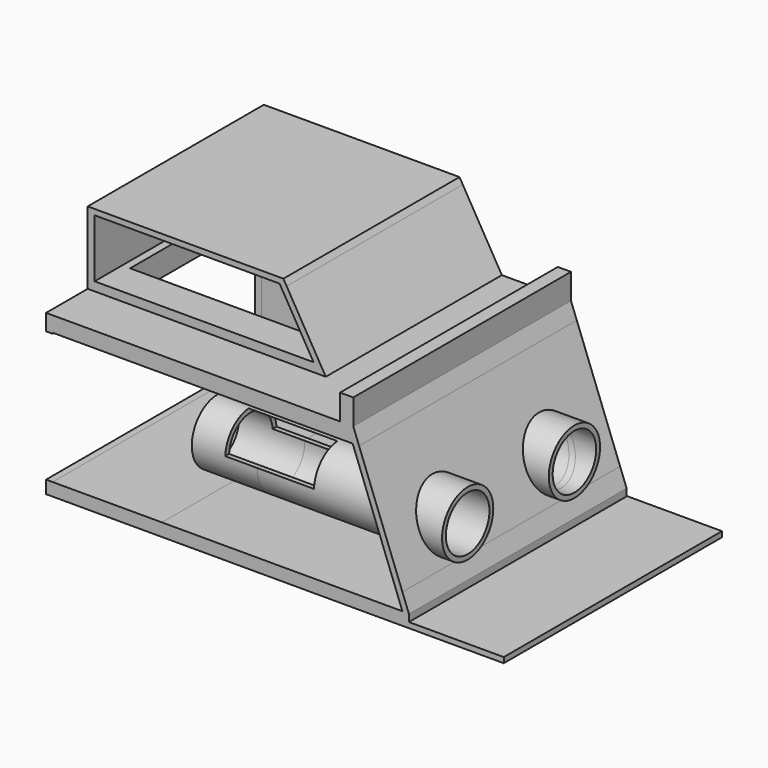
from build123d import *

# Parameters (mm, degrees)
F0_W      = 154.8604735136
F0_H      = 381
F0_W_2    = 202.8337074444
F0_W_3    = 150.305819042
F1_DEPTH  = 215.9
F3_DEPTH  = 365.76
F4_DEPTH  = 474.472
F5_DEPTH  = 384.81
F6_DEPTH  = 463.296
F7_DEPTH  = 453.644
F8_DEPTH  = 401.828
F9_W      = 333.3268084526
F9_H      = 308.1617667079
F10_DEPTH = 101.6
F12_DEPTH = 332.74
F13_DEPTH = 290.83
F14_W     = 640.7658
F14_H     = 381.7952661514
F15_DEPTH = 7.62
F16_W     = 18.4519021228
F16_H     = 174.1818501353
F16_H_2   = 32.6362997293
F17_DEPTH = 35.56
F18_R     = 44.8167953051
F18_R_2   = 38.1
F19_DEPTH = 258.572
F20_DEPTH = 485.14
F21_DEPTH = 258.572
F22_DEPTH = 57.658
F23_DEPTH = 72.898
F24_DEPTH = 250.19
F25_W     = 142.1934430047
F25_H     = 97.1279808664
F26_DEPTH = 68.58
F28_DEPTH = 340.868
F30_W     = 177.6428297162
F30_H     = 182.6925156638
F31_DEPTH = 723.9


# Not quite as in the source:
# - the program builds the solid bodies; features that only make, move or delete a surface that nothing else refers to are left out


with BuildPart() as f1:
    # F0 (on Top) → F1 (new body)
    with BuildSketch(Plane.XY):
        with Locations((-176.5697632432, 0)):
            Rectangle(F0_W, F0_H)
        with Locations((2.2773272358, 0)):
            Rectangle(F0_W_2, F0_H)
        with Locations((178.847090479, 0)):
            Rectangle(F0_W_3, F0_H)
    extrude(amount=F1_DEPTH)

    # F2 (on face) → F3 (cut)
    with BuildSketch(Plane.XZ.offset(190.5)):
        Polygon((-244.8522895575, 194.3728802726), (-244.8522895575, 10.3632332757), (244.8522895575, 10.3632332757), (175.2408137327, 194.3728802726), align=None)
    extrude(amount=-F3_DEPTH, mode=Mode.SUBTRACT)

    # F2 (on face) → F4 (cut)
    with BuildSketch(Plane.XZ.offset(190.5)):
        Polygon((215.0387168483, 194.3728802726), (244.8522895575, 115.5642510209), (244.8522895575, 194.3728802726), align=None)
    extrude(amount=-F4_DEPTH, mode=Mode.SUBTRACT)

    # F2 (on face) → F5 (cut)
    with BuildSketch(Plane.XZ.offset(190.5)):
        Polygon((244.8522895575, 194.3728802726), (244.8522895575, 115.5642510209), (254, 91.3833677769), (254, 215.9), (206.8949341774, 215.9), (215.0387168483, 194.3728802726), align=None)
    extrude(amount=-F5_DEPTH, mode=Mode.SUBTRACT)

    # F2 (on face) → F6 (cut)
    with BuildSketch(Plane.XZ.offset(190.5)):
        Polygon((184.2154591353, 194.3728802726), (244.8522895575, 34.0866396952), (244.8522895575, 115.5642510209), (215.0387168483, 194.3728802726), align=None)
    extrude(amount=-F6_DEPTH, mode=Mode.SUBTRACT)

    # F2 (on face) → F7 (cut)
    with BuildSketch(Plane.XZ.offset(190.5)):
        Polygon((244.8522895575, 115.5642510209), (244.8522895575, 34.0866396952), (254, 9.9057564512), (254, 91.3833677769), align=None)
    extrude(amount=-F7_DEPTH, mode=Mode.SUBTRACT)

    # F2 (on face) → F8 (cut)
    with BuildSketch(Plane.XZ.offset(190.5)):
        Polygon((176.0716764644, 215.9), (184.2154591353, 194.3728802726), (215.0387168483, 194.3728802726), (206.8949341774, 215.9), align=None)
    extrude(amount=-F8_DEPTH, mode=Mode.SUBTRACT)

    # F9 (on face) → F10 (join)
    with BuildSketch(Plane.XY.offset(215.9)):
        with Locations((-87.3365957737, 36.4191166461)):
            Rectangle(F9_W, F9_H)
    extrude(amount=F10_DEPTH)

    # F11 (on face) → F12 (cut)
    with BuildSketch(Plane.XZ.offset(117.6617667079)):
        Polygon((62.1921845761, 266.8175234586), (79.3268084526, 266.7), (79.3268084526, 317.5), (20.0025010854, 317.5), (24.5608866934, 309.6932172775), (62.1921845761, 309.6932172775), align=None)
        Polygon((62.1921845761, 245.2451009057), (79.3268084526, 215.9), (79.3268084526, 266.7), (62.1921845761, 266.8175234586), align=None)
        Polygon((24.5608866934, 309.6932172775), (49.5453838887, 266.9042657045), (62.1921845761, 266.8175234586), (62.1921845761, 309.6932172775), align=None)
        Polygon((49.5453838887, 266.9042657045), (62.1921845761, 245.2451009057), (62.1921845761, 266.8175234586), align=None)
    extrude(amount=-F12_DEPTH, mode=Mode.SUBTRACT)

    # F11 (on face) → F13 (cut)
    with BuildSketch(Plane.XZ.offset(117.6617667079)):
        Polygon((-87.3365957737, 267.843115824), (39.5991766547, 266.9724850411), (14.6545127754, 309.6932172775), (-87.3365957737, 309.6932172775), align=None)
        Polygon((-244.3442642689, 268.9200046058), (-87.3365957737, 267.843115824), (-87.3365957737, 309.6932172775), (-244.3442642689, 309.6932172775), align=None)
        Polygon((-87.3365957737, 228.2792460185), (62.1921845761, 228.2792460185), (39.5991766547, 266.9724850411), (-87.3365957737, 267.843115824), align=None)
        Polygon((-244.3442642689, 228.2792460185), (-87.3365957737, 228.2792460185), (-87.3365957737, 267.843115824), (-244.3442642689, 268.9200046058), align=None)
    extrude(amount=-F13_DEPTH, mode=Mode.SUBTRACT)

    # F14 (on face) → F15 (join)
    with BuildSketch(Plane(origin=(0, 0, 0), x_dir=(1, 0, 0), z_dir=(0, 0, -1))):
        with Locations((66.3829, -0.3976330757)):
            Rectangle(F14_W, F14_H)
    extrude(amount=F15_DEPTH)

    # F16 (on face) → F17 (join)
    with BuildSketch(Plane.XY.offset(215.9)):
        with Locations((166.845725403, 103.4090749323)):
            Rectangle(F16_W, F16_H)
        with Locations((166.845725403, 0)):
            Rectangle(F16_W, F16_H_2)
        with Locations((166.845725403, -103.4090749323)):
            Rectangle(F16_W, F16_H)
    extrude(amount=F17_DEPTH)

    # F18 (on Right) → F19 (join)
    with BuildSketch(Plane.YZ):
        with Locations((-93.4298427632, 83.6668761742)):
            Circle(F18_R)
        with Locations((-93.4298427632, 83.6668761742)):
            Circle(F18_R_2, mode=Mode.SUBTRACT)
    extrude(amount=F19_DEPTH)

    # F18 (on Right) → F20 (cut)
    with BuildSketch(Plane.YZ):
        with Locations((-93.4298427632, 83.6668761742)):
            Circle(F18_R_2)
    extrude(amount=F20_DEPTH, mode=Mode.SUBTRACT)

    # F18 (on Right) → F21 (join)
    with BuildSketch(Plane.YZ):
        with Locations((93.4298427632, 83.6668761742)):
            Circle(F18_R)
        with Locations((93.4298427632, 83.6668761742)):
            Circle(F18_R_2, mode=Mode.SUBTRACT)
        with Locations((-93.4298427632, 83.6668761742)):
            Circle(F18_R)
        with Locations((-93.4298427632, 83.6668761742)):
            Circle(F18_R_2, mode=Mode.SUBTRACT)
    extrude(amount=F21_DEPTH)

    # F18 (on Right) → F22 (cut)
    with BuildSketch(Plane.YZ):
        with Locations((-93.4298427632, 83.6668761742)):
            Circle(F18_R)
        with Locations((-93.4298427632, 83.6668761742)):
            Circle(F18_R_2, mode=Mode.SUBTRACT)
        with Locations((93.4298427632, 83.6668761742)):
            Circle(F18_R)
        with Locations((93.4298427632, 83.6668761742)):
            Circle(F18_R_2, mode=Mode.SUBTRACT)
    extrude(amount=-F22_DEPTH, mode=Mode.SUBTRACT)

    # F18 (on Right) + F21_face (on face) → F23 (cut)
    with BuildSketch(Plane.YZ):
        with Locations((-93.4298427632, 83.6668761742)):
            Circle(F18_R)
        with Locations((-93.4298427632, 83.6668761742)):
            Circle(F18_R_2, mode=Mode.SUBTRACT)
        with Locations((93.4298427632, 83.6668761742)):
            Circle(F18_R)
        with Locations((93.4298427632, 83.6668761742)):
            Circle(F18_R_2, mode=Mode.SUBTRACT)
    with BuildSketch(Plane(origin=(226.0959173271, 93.4298427632, 83.6668761742), x_dir=(0, 1, 0), z_dir=(0.9353094659, 0, 0.3538307547))):
        with BuildLine():
            add(Edge.make_bspline(
                [(38.1, 0), (38.1, -70.5554024353), (-19.05, -35.2777012177), (-76.2, 0), (-19.05, 35.2777012177), (38.1, 70.5554024353), (38.1, 0)],
                knots=[1.5707963268, 1.5707963268, 1.5707963268, 3.6651914292, 3.6651914292, 5.7595865316, 5.7595865316, 7.853981634, 7.853981634, 7.853981634], degree=2, weights=[1, 0.5, 1, 0.5, 1, 0.5, 1]))
        make_face()
    extrude(amount=-F23_DEPTH, dir=(1, 0, 0), mode=Mode.SUBTRACT)

    # F18 (on Right) → F24 (join)
    with BuildSketch(Plane.YZ):
        with Locations((-93.4298427632, 83.6668761742)):
            Circle(F18_R)
        with Locations((-93.4298427632, 83.6668761742)):
            Circle(F18_R_2, mode=Mode.SUBTRACT)
        with Locations((93.4298427632, 83.6668761742)):
            Circle(F18_R)
        with Locations((93.4298427632, 83.6668761742)):
            Circle(F18_R_2, mode=Mode.SUBTRACT)
    extrude(amount=-F24_DEPTH)

    # F25 (on face) → F26 (cut)
    with BuildSketch(Plane.XY.offset(228.2792460185)):
        with Locations((-162.1727613487, -20.8107571411)):
            Rectangle(F25_W, F25_H)
        with Locations((-19.979318344, -20.8107571411)):
            Rectangle(F25_W, F25_H)
        with Locations((-162.1727613487, 76.3172237253)):
            Rectangle(F25_W, F25_H)
        with Locations((-19.979318344, 76.3172237253)):
            Rectangle(F25_W, F25_H)
    extrude(amount=-F26_DEPTH, mode=Mode.SUBTRACT)

    # F27 (on face) → F28 (cut)
    with BuildSketch(Plane.XZ.offset(-175.26)):
        Polygon((-44.9973344803, 128.3188015223), (-44.9973344803, 85.9577953815), (79.164236784, 85.9577953815), (79.164236784, 121.7455416918), (79.164236784, 128.3188015223), align=None)
    extrude(amount=F28_DEPTH, mode=Mode.SUBTRACT)

    # F30 (on face) → F31 (cut)
    with BuildSketch(Plane.XZ.offset(-175.26)):
        with Locations((-180.61241135, 101.7094911076)):
            Rectangle(F30_W, F30_H)
    extrude(amount=F31_DEPTH, mode=Mode.SUBTRACT)


solid = f1.part
